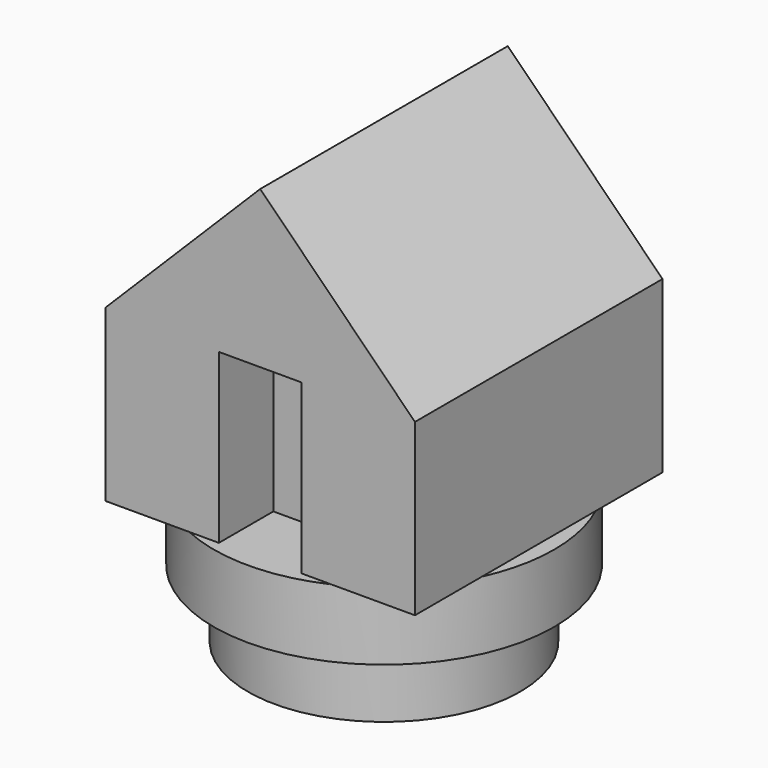
from build123d import *

# Parameters (mm, degrees)
F0_R        = 10.16
F1_DEPTH    = 5.08
F2_R        = 12.7
F2_R_2      = 10.16
F3_DEPTH    = 5.08
F5_DEPTH    = 25.4
F6_T1_DEPTH = 88.4028561312
F7_W        = 6.1679999344
F7_H        = 12.5403126109
F8_DEPTH    = 5.08


# Not quite as in the source:
# - a fillet or chamfer that OpenCascade refuses, or shapes differently, is made with other operations: its cross-section is extruded or revolved along the edge and cut away or added


with BuildPart() as f1:
    # F0 (on Top) → F1 (new body)
    with BuildSketch(Plane.XY):
        Circle(F0_R)
    extrude(amount=F1_DEPTH)

    # F2 (on face) → F3 (join)
    with BuildSketch(Plane.XY.offset(5.08)):
        Circle(F2_R)
        Circle(F2_R_2, mode=Mode.SUBTRACT)
        Circle(F2_R_2)
    extrude(amount=F3_DEPTH)

    # F4 (on face) → F5 (join)
    with BuildSketch(Plane.XY.offset(10.16)):
        with BuildLine():
            Line((-5.3003839328, -11.5410541184), (0, -11.5410541184))
            Line((0, -11.5410541184), (5.3003839328, -11.5410541184))
            ThreePointArc((5.3003839328, -11.5410541184), (7.254211996, -10.4243181224), (8.9802561211, -8.9802561211))
            ThreePointArc((8.9802561211, -8.9802561211), (10.4243181224, -7.254211996), (11.5410541184, -5.3003839328))
            Line((11.5410541184, -5.3003839328), (11.5410541184, 0))
            Line((11.5410541184, 0), (11.5410541184, 5.3003839328))
            ThreePointArc((11.5410541184, 5.3003839328), (8.9802561211, 8.9802561211), (5.3003839328, 11.5410541184))
            Line((5.3003839328, 11.5410541184), (-5.3003839328, 11.5410541184))
            ThreePointArc((-5.3003839328, 11.5410541184), (-8.9802561211, 8.9802561211), (-11.5410541184, 5.3003839328))
            Line((-11.5410541184, 5.3003839328), (-11.5410541184, -5.3003839328))
            ThreePointArc((-11.5410541184, -5.3003839328), (-8.9802561211, -8.9802561211), (-5.3003839328, -11.5410541184))
        make_face()
        with BuildLine():
            Line((-11.5410541184, -11.5410541184), (-5.3003839328, -11.5410541184))
            ThreePointArc((-5.3003839328, -11.5410541184), (-8.9802561211, -8.9802561211), (-11.5410541184, -5.3003839328))
            Line((-11.5410541184, -5.3003839328), (-11.5410541184, -11.5410541184))
        make_face()
        with BuildLine():
            Line((8.9802561211, -8.9802561211), (11.5410541184, -11.5410541184))
            Line((11.5410541184, -11.5410541184), (11.5410541184, -5.3003839328))
            ThreePointArc((11.5410541184, -5.3003839328), (10.4243181224, -7.254211996), (8.9802561211, -8.9802561211))
        make_face()
        with BuildLine():
            ThreePointArc((8.9802561211, -8.9802561211), (7.254211996, -10.4243181224), (5.3003839328, -11.5410541184))
            Line((5.3003839328, -11.5410541184), (11.5410541184, -11.5410541184))
            Line((11.5410541184, -11.5410541184), (8.9802561211, -8.9802561211))
        make_face()
        with BuildLine():
            Line((-11.5410541184, 11.5410541184), (-11.5410541184, 5.3003839328))
            ThreePointArc((-11.5410541184, 5.3003839328), (-8.9802561211, 8.9802561211), (-5.3003839328, 11.5410541184))
            Line((-5.3003839328, 11.5410541184), (-11.5410541184, 11.5410541184))
        make_face()
        with BuildLine():
            ThreePointArc((5.3003839328, 11.5410541184), (8.9802561211, 8.9802561211), (11.5410541184, 5.3003839328))
            Line((11.5410541184, 5.3003839328), (11.5410541184, 11.5410541184))
            Line((11.5410541184, 11.5410541184), (5.3003839328, 11.5410541184))
        make_face()
    extrude(amount=F5_DEPTH)

    # F6: chamfer of 12.7 on 2 edges, made by hand

    # F6_s2 → F6_t1 (cut)
    with BuildSketch(Plane.XZ.offset(-44.2014280656)):
        Polygon((11.5410541184, 22.86), (-1.1589458816, 35.56), (11.5410541184, 35.56), align=None)
        Polygon((-11.5410541184, 22.86), (1.1589458816, 35.56), (-11.5410541184, 35.56), align=None)
    extrude(amount=F6_T1_DEPTH, mode=Mode.SUBTRACT)

    # F7 (on face) → F8 (cut)
    with BuildSketch(Plane.XZ.offset(11.5410541184)):
        with Locations((0, 16.4301563054)):
            Rectangle(F7_W, F7_H)
    extrude(amount=-F8_DEPTH, mode=Mode.SUBTRACT)


solid = f1.part
